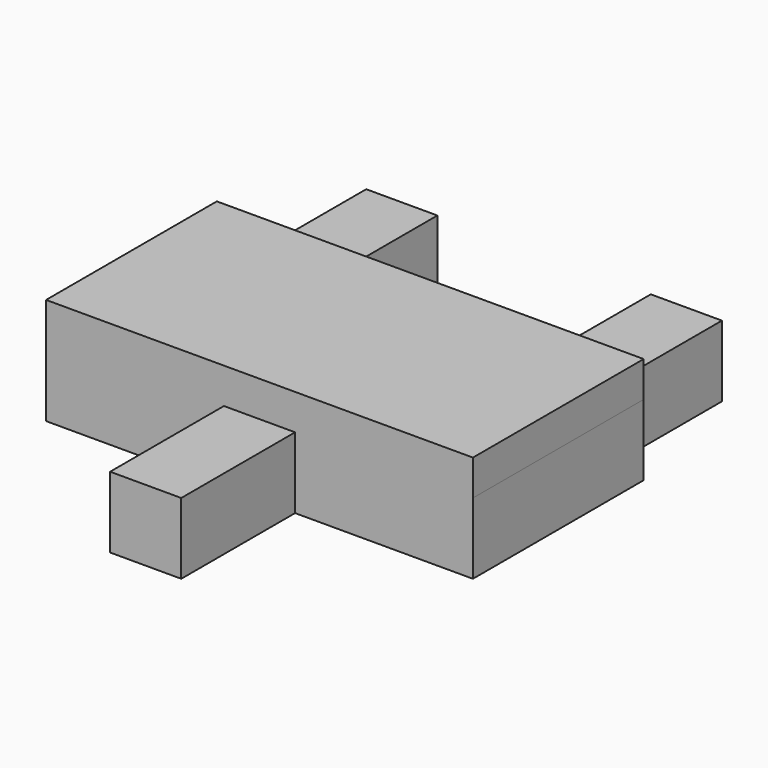
from build123d import *

# Parameters (mm, degrees)
F0_W     = 0.508
F0_H     = 1.016
F1_DEPTH = 0.762
F2_W     = 5.1749609411
F2_H     = 4.1793081909
F2_W_2   = 3.0479989649
F2_H_2   = 1.524
F3_DEPTH = 0.254


# Not quite as in the source:
# - ends of sketch curves that miss each other by under 0.0002 mm in the source are joined


with BuildPart() as f1:
    # F0 (on Top) → F1 (new body)
    with BuildSketch(Plane.XY):
        Polygon((-1.27, 0.762), (-1.524, 0.762), (-1.524, -0.762), (-0.254, -0.762), (0.254, -0.762), (1.524, -0.762), (1.524, 0.762), (1.27, 0.762), (0.762, 0.762), (-0.762, 0.762), align=None)
        with Locations((-1.016, 1.27)):
            Rectangle(F0_W, F0_H)
        with Locations((0, -1.27)):
            Rectangle(F0_W, F0_H)
        Polygon((0.762, 1.7779941872), (0.762, 0.7619941872), (1.27, 0.762), (1.27, 1.7779941872), align=None)
    extrude(amount=F1_DEPTH)

    # F2 (on face) → F3 (cut)
    with BuildSketch(Plane.XY.offset(0.762)):
        Rectangle(F2_W, F2_H)
        Rectangle(F2_W_2, F2_H_2, mode=Mode.SUBTRACT)
    extrude(amount=-F3_DEPTH, mode=Mode.SUBTRACT)


solid = f1.part
